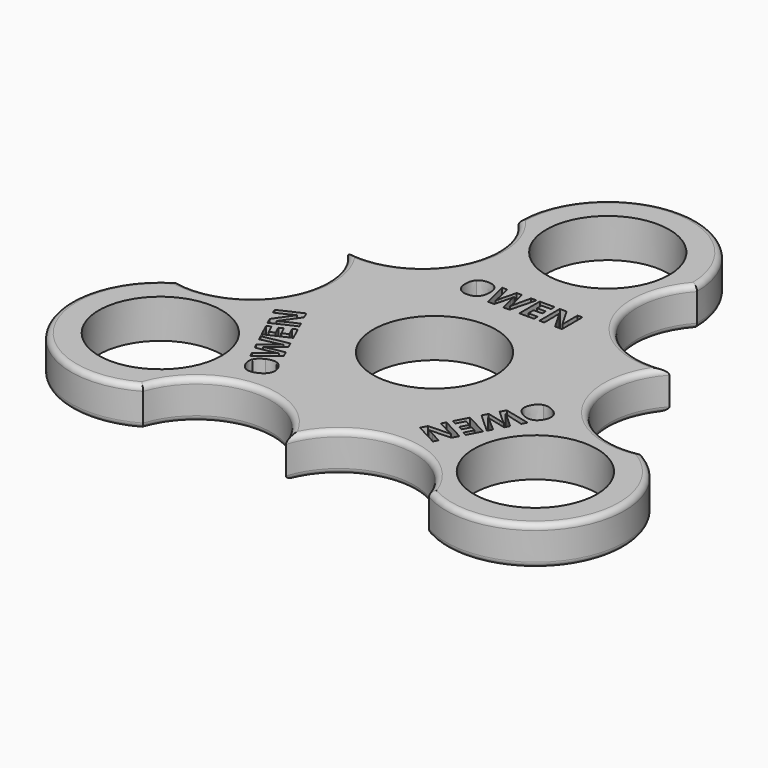
from build123d import *

# Parameters (mm, degrees)
F0_R     = 11.05
F1_DEPTH = 7
F2_R     = 1


# Not quite as in the source:
# - ends of sketch curves that miss each other by under 0.0002 mm in the source are joined


with BuildPart() as f1:
    # F0 (on Top) → F1 (new body)
    with BuildSketch(Plane.XY):
        with BuildLine():
            ThreePointArc((28.9033447387, 16.6873538654), (14.3582929081, 23.1315283654), (16.05, 38.95))
            ThreePointArc((16.05, 38.95), (0, 55), (-16.05, 38.95))
            ThreePointArc((-16.05, 38.95), (-14.3582932677, 23.1315285729), (-28.9033450982, 16.6873540729))
            ThreePointArc((-28.9033450982, 16.6873540729), (-27.2116376469, 0.8688822307), (-41.7566894774, -5.5752922693))
            ThreePointArc((-41.7566894774, -5.5752922693), (-47.6313972081, -27.5), (-25.7066894774, -33.3747077307))
            ThreePointArc((-25.7066894774, -33.3747077307), (-12.8533447387, -24.0004110112), (0, -33.3747081459))
            ThreePointArc((0, -33.3747081459), (12.8533447387, -24.0004105961), (25.7066894774, -33.3747077307))
            ThreePointArc((25.7066894774, -33.3747077307), (47.6313972081, -27.5), (41.7566894774, -5.5752922693))
            ThreePointArc((41.7566894774, -5.5752922693), (27.2116380064, 0.8688824383), (28.9033447387, 16.6873538654))
        make_face()
        with Locations((-33.7316894774, -19.475)):
            Circle(F0_R, mode=Mode.SUBTRACT)
        with BuildLine():
            Line((-22.1243997237, -11.4330353899), (-17.47080053, -10.5521203449))
            Line((-17.47080053, -10.5521203449), (-17.0025219196, -11.5563470656))
            Line((-17.0025219196, -11.5563470656), (-18.9248062984, -13.1388357374))
            add(Edge.make_bspline(
                [(-18.9248062984, -13.1388357374), (-19.0269092426, -13.2241334442), (-19.3572174055, -13.4701576327)],
                knots=[0, 0, 0, 1, 1, 1], degree=2))
            add(Edge.make_bspline(
                [(-19.3572174055, -13.4701576327), (-19.6875255684, -13.7161818212), (-19.8080731152, -13.7856951202)],
                knots=[0, 0, 0, 1, 1, 1], degree=2))
            add(Edge.make_bspline(
                [(-19.8080731152, -13.7856951202), (-19.6461405591, -13.7312447327), (-19.2742461113, -13.6409590963)],
                knots=[0, 0, 0, 1, 1, 1], degree=2))
            add(Edge.make_bspline(
                [(-19.2742461113, -13.6409590963), (-18.9023516635, -13.5506734599), (-18.7401835115, -13.5204984794)],
                knots=[0, 0, 0, 1, 1, 1], degree=2))
            Line((-18.7401835115, -13.5204984794), (-16.2994671791, -13.0640528221))
            Line((-16.2994671791, -13.0640528221), (-15.8324622186, -14.0655481918))
            Line((-15.8324622186, -14.0655481918), (-19.497284546, -17.0669020695))
            Line((-19.497284546, -17.0669020695), (-19.9018806617, -16.1992428992))
            Line((-19.9018806617, -16.1992428992), (-17.8795792526, -14.6078018422))
            add(Edge.make_bspline(
                [(-17.8795792526, -14.6078018422), (-17.3154142148, -14.1751389156), (-16.8835957424, -13.898406011)],
                knots=[0, 0, 0, 1, 1, 1], degree=2))
            add(Edge.make_bspline(
                [(-16.8835957424, -13.898406011), (-17.0537223515, -13.9566773482), (-17.4224326746, -14.0537913621)],
                knots=[0, 0, 0, 1, 1, 1], degree=2))
            add(Edge.make_bspline(
                [(-17.4224326746, -14.0537913621), (-17.7911429977, -14.150905376), (-18.0037442148, -14.1846460987)],
                knots=[0, 0, 0, 1, 1, 1], degree=2))
            Line((-18.0037442148, -14.1846460987), (-20.6172473512, -14.665134083))
            Line((-20.6172473512, -14.665134083), (-21.0057105683, -13.8320720255))
            Line((-21.0057105683, -13.8320720255), (-18.9577079841, -12.1388641936))
            add(Edge.make_bspline(
                [(-18.9577079841, -12.1388641936), (-18.820701175, -12.026206335), (-18.5266650039, -11.8164934256)],
                knots=[0, 0, 0, 1, 1, 1], degree=2))
            add(Edge.make_bspline(
                [(-18.5266650039, -11.8164934256), (-18.2326288327, -11.6067805163), (-18.0167195965, -11.468414064)],
                knots=[0, 0, 0, 1, 1, 1], degree=2))
            add(Edge.make_bspline(
                [(-18.0167195965, -11.468414064), (-18.2520305274, -11.5437802948), (-18.6127283972, -11.6354954085)],
                knots=[0, 0, 0, 1, 1, 1], degree=2))
            add(Edge.make_bspline(
                [(-18.6127283972, -11.6354954085), (-18.9734262671, -11.7272105223), (-19.2020523907, -11.7717490454)],
                knots=[0, 0, 0, 1, 1, 1], degree=2))
            Line((-19.2020523907, -11.7717490454), (-21.7193790579, -12.3016050105))
            Line((-21.7193790579, -12.3016050105), (-22.1243997237, -11.4330353899))
        make_face(mode=Mode.SUBTRACT)
        with BuildLine():
            add(Edge.make_bspline(
                [(-18.6158173747, -17.6866989262), (-18.3005281259, -16.9211780855), (-17.2653460938, -16.4384647764)],
                knots=[0, 0, 0, 1, 1, 1], degree=2))
            add(Edge.make_bspline(
                [(-17.2653460938, -16.4384647764), (-16.2319849623, -15.9566005671), (-15.4382561277, -16.2099656781)],
                knots=[0, 0, 0, 1, 1, 1], degree=2))
            add(Edge.make_bspline(
                [(-15.4382561277, -16.2099656781), (-14.6445272931, -16.463330789), (-14.1987498308, -17.4193036419)],
                knots=[0, 0, 0, 1, 1, 1], degree=2))
            add(Edge.make_bspline(
                [(-14.1987498308, -17.4193036419), (-13.7529723685, -18.3752764947), (-14.0690824936, -19.1461680119)],
                knots=[0, 0, 0, 1, 1, 1], degree=2))
            add(Edge.make_bspline(
                [(-14.0690824936, -19.1461680119), (-14.3851926186, -19.917059529), (-15.424016452, -20.401471038)],
                knots=[0, 0, 0, 1, 1, 1], degree=2))
            add(Edge.make_bspline(
                [(-15.424016452, -20.401471038), (-16.4628402855, -20.885882547), (-17.2499223424, -20.6277553609)],
                knots=[0, 0, 0, 1, 1, 1], degree=2))
            add(Edge.make_bspline(
                [(-17.2499223424, -20.6277553609), (-18.0370043993, -20.3696281747), (-18.4840555114, -19.4109239709)],
                knots=[0, 0, 0, 1, 1, 1], degree=2))
            add(Edge.make_bspline(
                [(-18.4840555114, -19.4109239709), (-18.9311066236, -18.452219767), (-18.6158173747, -17.6866989262)],
                knots=[0, 0, 0, 1, 1, 1], degree=2))
        make_face(mode=Mode.SUBTRACT)
        Polygon((-20.0540195919, -6.9140027979), (-19.325659323, -6.5743628266), (-18.2086683675, -8.9697576608), (-22.368515953, -10.9095264467), (-23.4855069085, -8.5141316125), (-22.7626093417, -8.177038941), (-22.0570073014, -9.6902073996), (-21.1438256143, -9.2643837856), (-21.8006044087, -7.8559171157), (-21.0777068419, -7.5188244442), (-20.4209280475, -8.9272911141), (-19.3484175516, -8.4271712564), align=None, mode=Mode.SUBTRACT)
        with BuildLine():
            Line((-25.6108040287, -3.9564172302), (-21.4509564432, -2.0166484443))
            Line((-21.4509564432, -2.0166484443), (-20.9283354374, -3.137412808))
            Line((-20.9283354374, -3.137412808), (-23.2308464703, -6.4146327519))
            Line((-23.2308464703, -6.4146327519), (-23.2189590713, -6.4401253613))
            add(Edge.make_bspline(
                [(-23.2189590713, -6.4401253613), (-22.4113700116, -5.9970351241), (-22.0553839302, -5.8310360881)],
                knots=[0, 0, 0, 1, 1, 1], degree=2))
            Line((-22.0553839302, -5.8310360881), (-20.0979157077, -4.9182536653))
            Line((-20.0979157077, -4.9182536653), (-19.7302554388, -5.7067036564))
            Line((-19.7302554388, -5.7067036564), (-23.8901030243, -7.6464724422))
            Line((-23.8901030243, -7.6464724422), (-24.4089030804, -6.5339021316))
            Line((-24.4089030804, -6.5339021316), (-22.1356491591, -3.2747586877))
            Line((-22.1356491591, -3.2747586877), (-22.1449892583, -3.2547287803))
            add(Edge.make_bspline(
                [(-22.1449892583, -3.2547287803), (-22.9362466594, -3.6757939641), (-23.2712923831, -3.8320283509)],
                knots=[0, 0, 0, 1, 1, 1], degree=2))
            Line((-23.2712923831, -3.8320283509), (-25.24059646, -4.7503299232))
            Line((-25.24059646, -4.7503299232), (-25.6108040287, -3.9564172302))
        make_face(mode=Mode.SUBTRACT)
        with BuildLine():
            Line((16.7794067216, -21.3347600573), (12.7262140445, -19.1810042681))
            Line((12.7262140445, -19.1810042681), (13.3064883664, -18.0889753371))
            Line((13.3064883664, -18.0889753371), (17.3094431488, -17.9545111143))
            Line((17.3094431488, -17.9545111143), (17.3226419149, -17.9296721134))
            add(Edge.make_bspline(
                [(17.3226419149, -17.9296721134), (16.4826557807, -17.5515817246), (16.1357968758, -17.3672703843)],
                knots=[0, 0, 0, 1, 1, 1], degree=2))
            Line((16.1357968758, -17.3672703843), (14.2285164521, -16.3537937052))
            Line((14.2285164521, -16.3537937052), (14.6367354308, -15.5855588927))
            Line((14.6367354308, -15.5855588927), (18.6899281079, -17.739314682))
            Line((18.6899281079, -17.739314682), (18.1138962465, -18.8233596483))
            Line((18.1138962465, -18.8233596483), (14.142988646, -18.9703025156))
            Line((14.142988646, -18.9703025156), (14.1326181869, -18.9898188734))
            add(Edge.make_bspline(
                [(14.1326181869, -18.9898188734), (14.9451857504, -19.3681284274), (15.2716411903, -19.5415979241)],
                knots=[0, 0, 0, 1, 1, 1], degree=2))
            Line((15.2716411903, -19.5415979241), (17.1904540072, -20.5612026018))
            Line((17.1904540072, -20.5612026018), (16.7794067216, -21.3347600573))
        make_face(mode=Mode.SUBTRACT)
        Polygon((15.7956506002, -15.1172533576), (15.0859648611, -14.7401457561), (16.3261774857, -12.4061667818), (20.3793701627, -14.5599225711), (19.1391575382, -16.8939015453), (18.4347944422, -16.5196222508), (19.2182354844, -15.045250128), (18.3284669891, -14.5724514725), (17.5992351646, -15.9448062704), (16.8948720686, -15.5705269759), (17.6241038931, -14.198172178), (16.5790916424, -13.6428812348), align=None, mode=Mode.SUBTRACT)
        with Locations((33.7316894774, -19.475)):
            Circle(F0_R, mode=Mode.SUBTRACT)
        with BuildLine():
            Line((20.6504162513, -14.0498359462), (17.14544375, -10.8643745138))
            Line((17.14544375, -10.8643745138), (17.6653808556, -9.8858953011))
            Line((17.6653808556, -9.8858953011), (20.0862250794, -10.4680987651))
            add(Edge.make_bspline(
                [(20.0862250794, -10.4680987651), (20.2158018707, -10.4982743374), (20.6111003147, -10.6139053195)],
                knots=[0, 0, 0, 1, 1, 1], degree=2))
            add(Edge.make_bspline(
                [(20.6111003147, -10.6139053195), (21.0063987586, -10.7295363016), (21.1344761626, -10.7839420768)],
                knots=[0, 0, 0, 1, 1, 1], degree=2))
            add(Edge.make_bspline(
                [(21.1344761626, -10.7839420768), (20.9935113558, -10.6874230597), (20.697530664, -10.4448279102)],
                knots=[0, 0, 0, 1, 1, 1], degree=2))
            add(Edge.make_bspline(
                [(20.697530664, -10.4448279102), (20.4015499722, -10.2022327607), (20.2798266962, -10.0909112308)],
                knots=[0, 0, 0, 1, 1, 1], degree=2))
            Line((20.2798266962, -10.0909112308), (18.4459935908, -8.4168458213))
            Line((18.4459935908, -8.4168458213), (18.9645165429, -7.4410279301))
            Line((18.9645165429, -7.4410279301), (23.5673435492, -8.5604167547))
            Line((23.5673435492, -8.5604167547), (23.1181141189, -9.4058298914))
            Line((23.1181141189, -9.4058298914), (20.6299088938, -8.7491546402))
            add(Edge.make_bspline(
                [(20.6299088938, -8.7491546402), (19.944796008, -8.559155347), (19.4638656319, -8.3809580769)],
                knots=[0, 0, 0, 1, 1, 1], degree=2))
            add(Edge.make_bspline(
                [(19.4638656319, -8.3809580769), (19.6128144033, -8.4817195545), (19.9123304788, -8.7176614002)],
                knots=[0, 0, 0, 1, 1, 1], degree=2))
            add(Edge.make_bspline(
                [(19.9123304788, -8.7176614002), (20.2118465543, -8.9536032459), (20.3667789465, -9.1030477765)],
                knots=[0, 0, 0, 1, 1, 1], degree=2))
            Line((20.3667789465, -9.1030477765), (22.3238312332, -10.9006054792))
            Line((22.3238312332, -10.9006054792), (21.8925144139, -11.7123085432))
            Line((21.8925144139, -11.7123085432), (19.3075779707, -11.0963775961))
            add(Edge.make_bspline(
                [(19.3075779707, -11.0963775961), (19.1351417259, -11.0548035619), (18.7906736551, -10.9462746603)],
                knots=[0, 0, 0, 1, 1, 1], degree=2))
            add(Edge.make_bspline(
                [(18.7906736551, -10.9462746603), (18.4462055843, -10.8377457588), (18.2057403963, -10.7486471237)],
                knots=[0, 0, 0, 1, 1, 1], degree=2))
            add(Edge.make_bspline(
                [(18.2057403963, -10.7486471237), (18.4075816271, -10.8911652646), (18.6979631077, -11.1239596182)],
                knots=[0, 0, 0, 1, 1, 1], degree=2))
            add(Edge.make_bspline(
                [(18.6979631077, -11.1239596182), (18.9883445884, -11.3567539719), (19.1615461704, -11.5124934866)],
                knots=[0, 0, 0, 1, 1, 1], degree=2))
            Line((19.1615461704, -11.5124934866), (21.1001170662, -13.2035357024))
            Line((21.1001170662, -13.2035357024), (20.6504162513, -14.0498359462))
        make_face(mode=Mode.SUBTRACT)
        with BuildLine():
            add(Edge.make_bspline(
                [(23.5315723516, -7.4834520668), (22.7305092986, -7.6925631694), (21.721868442, -7.1565989907)],
                knots=[0, 0, 0, 1, 1, 1], degree=2))
            add(Edge.make_bspline(
                [(21.721868442, -7.1565989907), (20.7150017998, -6.621577581), (20.4394637597, -5.8352709419)],
                knots=[0, 0, 0, 1, 1, 1], degree=2))
            add(Edge.make_bspline(
                [(20.4394637597, -5.8352709419), (20.1639257196, -5.0489643027), (20.6588794466, -4.1175017702)],
                knots=[0, 0, 0, 1, 1, 1], degree=2))
            add(Edge.make_bspline(
                [(20.6588794466, -4.1175017702), (21.1538331736, -3.1860392377), (21.9596787784, -2.9743503064)],
                knots=[0, 0, 0, 1, 1, 1], degree=2))
            add(Edge.make_bspline(
                [(21.9596787784, -2.9743503064), (22.7655243831, -2.7626613751), (23.7777136684, -3.3005110917)],
                knots=[0, 0, 0, 1, 1, 1], degree=2))
            add(Edge.make_bspline(
                [(23.7777136684, -3.3005110917), (24.7899029537, -3.8383608084), (25.0576370597, -4.6222270324)],
                knots=[0, 0, 0, 1, 1, 1], degree=2))
            add(Edge.make_bspline(
                [(25.0576370597, -4.6222270324), (25.3253711656, -5.4060932563), (24.8290032851, -6.3402171103)],
                knots=[0, 0, 0, 1, 1, 1], degree=2))
            add(Edge.make_bspline(
                [(24.8290032851, -6.3402171103), (24.3326354046, -7.2743409643), (23.5315723516, -7.4834520668)],
                knots=[0, 0, 0, 1, 1, 1], degree=2))
        make_face(mode=Mode.SUBTRACT)
        Circle(F0_R, mode=Mode.SUBTRACT)
        with BuildLine():
            add(Edge.make_bspline(
                [(-5.8169672008, 20.7402947464), (-5.256416696, 20.1310225579), (-5.256416696, 18.9888255616)],
                knots=[0, 0, 0, 1, 1, 1], degree=2))
            add(Edge.make_bspline(
                [(-5.256416696, 18.9888255616), (-5.256416696, 17.8486377068), (-5.8214877694, 17.236351806)],
                knots=[0, 0, 0, 1, 1, 1], degree=2))
            add(Edge.make_bspline(
                [(-5.8214877694, 17.236351806), (-6.3865588427, 16.6240659052), (-7.4413581797, 16.6240659052)],
                knots=[0, 0, 0, 1, 1, 1], degree=2))
            add(Edge.make_bspline(
                [(-7.4413581797, 16.6240659052), (-8.4961575167, 16.6240659052), (-9.0612285901, 17.236351806)],
                knots=[0, 0, 0, 1, 1, 1], degree=2))
            add(Edge.make_bspline(
                [(-9.0612285901, 17.236351806), (-9.6262996635, 17.8486377068), (-9.6262996635, 18.9948529864)],
                knots=[0, 0, 0, 1, 1, 1], degree=2))
            add(Edge.make_bspline(
                [(-9.6262996635, 18.9948529864), (-9.6262996635, 20.1410682659), (-9.0597217339, 20.7453176004)],
                knots=[0, 0, 0, 1, 1, 1], degree=2))
            add(Edge.make_bspline(
                [(-9.0597217339, 20.7453176004), (-8.4931438043, 21.3495669348), (-7.4353307549, 21.3495669348)],
                knots=[0, 0, 0, 1, 1, 1], degree=2))
            add(Edge.make_bspline(
                [(-7.4353307549, 21.3495669348), (-6.3775177056, 21.3495669348), (-5.8169672008, 20.7402947464)],
                knots=[0, 0, 0, 1, 1, 1], degree=2))
        make_face(mode=Mode.SUBTRACT)
        with BuildLine():
            Line((1.3335677332, 21.2772378374), (0.1652518961, 16.6873538654))
            Line((0.1652518961, 16.6873538654), (-0.9427896931, 16.6873538654))
            Line((-0.9427896931, 16.6873538654), (-1.5646190165, 19.0983237785))
            add(Edge.make_bspline(
                [(-1.5646190165, 19.0983237785), (-1.5987744236, 19.2269088405), (-1.6821537998, 19.6302440156)],
                knots=[0, 0, 0, 1, 1, 1], degree=2))
            add(Edge.make_bspline(
                [(-1.6821537998, 19.6302440156), (-1.765533176, 20.0335791906), (-1.7775880255, 20.1722099606)],
                knots=[0, 0, 0, 1, 1, 1], degree=2))
            add(Edge.make_bspline(
                [(-1.7775880255, 20.1722099606), (-1.7966748707, 20.0024374959), (-1.8720176804, 19.6272303032)],
                knots=[0, 0, 0, 1, 1, 1], degree=2))
            add(Edge.make_bspline(
                [(-1.8720176804, 19.6272303032), (-1.9473604902, 19.2520231104), (-1.9885478929, 19.0922963537)],
                knots=[0, 0, 0, 1, 1, 1], degree=2))
            Line((-1.9885478929, 19.0922963537), (-2.6063589331, 16.6873538654))
            Line((-2.6063589331, 16.6873538654), (-3.71138681, 16.6873538654))
            Line((-3.71138681, 16.6873538654), (-4.8827163594, 21.2772378374))
            Line((-4.8827163594, 21.2772378374), (-3.9253603898, 21.2772378374))
            Line((-3.9253603898, 21.2772378374), (-3.3376864735, 18.7718382694))
            add(Edge.make_bspline(
                [(-3.3376864735, 18.7718382694), (-3.1839871415, 18.0776798486), (-3.1156763273, 17.5693670252)],
                knots=[0, 0, 0, 1, 1, 1], degree=2))
            add(Edge.make_bspline(
                [(-3.1156763273, 17.5693670252), (-3.0965894821, 17.7481806271), (-3.0287809533, 18.1233878199)],
                knots=[0, 0, 0, 1, 1, 1], degree=2))
            add(Edge.make_bspline(
                [(-3.0287809533, 18.1233878199), (-2.9609724245, 18.4985950126), (-2.9017027475, 18.7055365968)],
                knots=[0, 0, 0, 1, 1, 1], degree=2))
            Line((-2.9017027475, 18.7055365968), (-2.2326585966, 21.2772378374))
            Line((-2.2326585966, 21.2772378374), (-1.3134763172, 21.2772378374))
            Line((-1.3134763172, 21.2772378374), (-0.6444321664, 18.7055365968))
            add(Edge.make_bspline(
                [(-0.6444321664, 18.7055365968), (-0.6002310513, 18.5337549905), (-0.5344316641, 18.1786392137)],
                knots=[0, 0, 0, 1, 1, 1], degree=2))
            add(Edge.make_bspline(
                [(-0.5344316641, 18.1786392137), (-0.4686322769, 17.8235234369), (-0.4344768698, 17.5693670252)],
                knots=[0, 0, 0, 1, 1, 1], degree=2))
            add(Edge.make_bspline(
                [(-0.4344768698, 17.5693670252), (-0.403335175, 17.8144822997), (-0.33401979, 18.1801460699)],
                knots=[0, 0, 0, 1, 1, 1], degree=2))
            add(Edge.make_bspline(
                [(-0.33401979, 18.1801460699), (-0.264704405, 18.5458098401), (-0.2084484404, 18.7718382694)],
                knots=[0, 0, 0, 1, 1, 1], degree=2))
            Line((-0.2084484404, 18.7718382694), (0.3752071927, 21.2772378374))
            Line((0.3752071927, 21.2772378374), (1.3335677332, 21.2772378374))
        make_face(mode=Mode.SUBTRACT)
        Polygon((4.5542217088, 17.4910105031), (4.5542217088, 16.6873538654), (1.9111959415, 16.6873538654), (1.9111959415, 21.2772378374), (4.5542217088, 21.2772378374), (4.5542217088, 20.4796086245), (2.8846250439, 20.4796086245), (2.8846250439, 19.472024115), (4.4386960671, 19.472024115), (4.4386960671, 18.6743949021), (2.8846250439, 18.6743949021), (2.8846250439, 17.4910105031), align=None, mode=Mode.SUBTRACT)
        with BuildLine():
            Line((9.5831031192, 21.2772378374), (9.5831031192, 16.6873538654))
            Line((9.5831031192, 16.6873538654), (8.3464764679, 16.6873538654))
            Line((8.3464764679, 16.6873538654), (6.3493897232, 20.1591505402))
            Line((6.3493897232, 20.1591505402), (6.3212617409, 20.1591505402))
            add(Edge.make_bspline(
                [(6.3212617409, 20.1591505402), (6.3815359887, 19.2399682609), (6.3815359887, 18.8471810792)],
                knots=[0, 0, 0, 1, 1, 1], degree=2))
            Line((6.3815359887, 18.8471810792), (6.3815359887, 16.6873538654))
            Line((6.3815359887, 16.6873538654), (5.5115776784, 16.6873538654))
            Line((5.5115776784, 16.6873538654), (5.5115776784, 21.2772378374))
            Line((5.5115776784, 21.2772378374), (6.7391631925, 21.2772378374))
            Line((6.7391631925, 21.2772378374), (8.732231654, 17.8395965697))
            Line((8.732231654, 17.8395965697), (8.7543322116, 17.8395965697))
            add(Edge.make_bspline(
                [(8.7543322116, 17.8395965697), (8.7071173841, 18.7346691499), (8.7071173841, 19.1043512033)],
                knots=[0, 0, 0, 1, 1, 1], degree=2))
            Line((8.7071173841, 19.1043512033), (8.7071173841, 21.2772378374))
            Line((8.7071173841, 21.2772378374), (9.5831031192, 21.2772378374))
        make_face(mode=Mode.SUBTRACT)
        with Locations((0, 38.95)):
            Circle(F0_R, mode=Mode.SUBTRACT)
    extrude(amount=F1_DEPTH)

    # F2
    f2_edges = [f1.edges().sort_by_distance(p)[0] for p in [
        (-14.358293, 23.131528, 7),
        (0, 55, 7),
        (14.358293, 23.131528, 7),
        (27.211638, 0.868882, 7),
        (47.631397, -27.5, 7),
        (12.853345, -24.000411, 7),
        (-12.853345, -24.000411, 7),
        (-27.211638, 0.868882, 7),
        (-47.631397, -27.5, 7),
        (-12.853345, -24.000411, 0),
        (-47.631397, -27.5, 0),
        (-27.211638, 0.868882, 0),
        (-14.358293, 23.131528, 0),
        (0, 55, 0),
        (14.358293, 23.131528, 0),
        (27.211638, 0.868882, 0),
        (47.631397, -27.5, 0),
        (12.853345, -24.000411, 0),
    ]]
    fillet(f2_edges, radius=F2_R)


solid = f1.part
